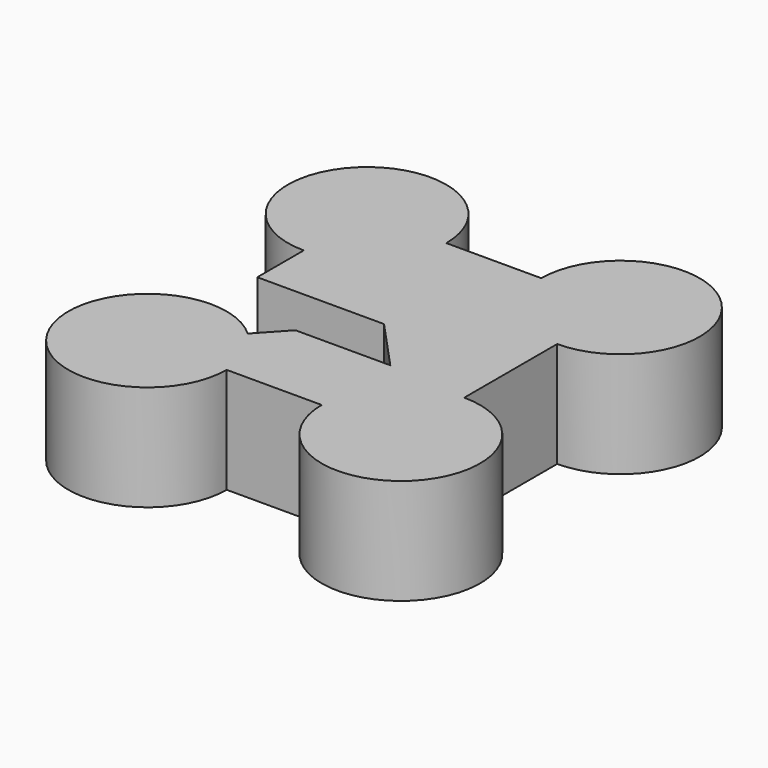
from build123d import *

# Parameters (mm, degrees)
F1_DEPTH = 25.4


with BuildPart() as f1:
    # F0 (on Top) → F1 (new body)
    with BuildSketch(Plane.XY):
        with BuildLine():
            Line((-30.48, 13.97), (-30.48, 0))
            Line((-30.48, 0), (-11.4207109466, 0))
            Line((-11.4207109466, 0), (-11.4207109466, 12.3724368588))
            Line((-11.4207109466, 12.3724368588), (-17.5587640429, 19.0219943798))
            ThreePointArc((-17.5587640429, 19.0219943798), (-23.5431241565, 15.277896023), (-30.48, 13.97))
        make_face()
        Polygon((-11.4207109466, 12.3724368588), (-11.4207109466, 0), (0, 0), align=None)
        with BuildLine():
            ThreePointArc((-17.5587640429, -19.0219943798), (-23.5431241565, -15.277896023), (-30.48, -13.97))
            Line((-30.48, -13.97), (-30.48, -33.02))
            Line((-30.48, -33.02), (-17.5587640429, -19.0219943798))
        make_face()
        with BuildLine():
            Line((-30.48, -33.02), (-30.48, -13.97))
            ThreePointArc((-30.48, -13.97), (-43.9503841816, -46.4903841816), (-11.43, -33.02))
            Line((-11.43, -33.02), (-30.48, -33.02))
        make_face()
        with BuildLine():
            ThreePointArc((-49.53, 33.02), (-43.9503841816, 19.5496158184), (-30.48, 13.97))
            Line((-30.48, 13.97), (-30.48, 33.02))
            Line((-30.48, 33.02), (-49.53, 33.02))
        make_face()
        with BuildLine():
            Line((-30.48, 33.02), (-30.48, 13.97))
            ThreePointArc((-30.48, 13.97), (-23.5431241565, 15.277896023), (-17.5587640429, 19.0219943798))
            Line((-17.5587640429, 19.0219943798), (-30.48, 33.02))
        make_face()
        Polygon((11.4207109466, 12.3724368588), (0, 0), (11.4207109466, 0), align=None)
        Polygon((-11.4207109466, 12.3724368588), (0, 0), (11.4207109466, 12.3724368588), align=None)
        Polygon((11.4207109466, 0), (0, 0), (11.4207109466, -12.3724368588), align=None)
        with BuildLine():
            Line((-17.5587640429, 19.0219943798), (-11.4207109466, 12.3724368588))
            Line((-11.4207109466, 12.3724368588), (11.4207109466, 12.3724368588))
            Line((11.4207109466, 12.3724368588), (17.5587640429, 19.0219943798))
            ThreePointArc((17.5587640429, 19.0219943798), (13.0293260161, 25.3795499145), (11.43, 33.02))
            Line((11.43, 33.02), (-11.43, 33.02))
            ThreePointArc((-11.43, 33.02), (-13.0293260161, 25.3795499145), (-17.5587640429, 19.0219943798))
        make_face()
        with BuildLine():
            Line((11.4207109466, -12.3724368588), (-11.4207109466, -12.3724368588))
            Line((-11.4207109466, -12.3724368588), (-17.5587640429, -19.0219943798))
            ThreePointArc((-17.5587640429, -19.0219943798), (-13.0293260161, -25.3795499145), (-11.43, -33.02))
            Line((-11.43, -33.02), (11.43, -33.02))
            ThreePointArc((11.43, -33.02), (13.0293260161, -25.3795499145), (17.5587640429, -19.0219943798))
            Line((17.5587640429, -19.0219943798), (11.4207109466, -12.3724368588))
        make_face()
        with BuildLine():
            Line((-17.5587640429, -19.0219943798), (-30.48, -33.02))
            Line((-30.48, -33.02), (-11.43, -33.02))
            ThreePointArc((-11.43, -33.02), (-13.0293260161, -25.3795499145), (-17.5587640429, -19.0219943798))
        make_face()
        with BuildLine():
            Line((-49.53, 33.02), (-30.48, 33.02))
            Line((-30.48, 33.02), (-11.43, 33.02))
            ThreePointArc((-11.43, 33.02), (-30.48, 52.07), (-49.53, 33.02))
        make_face()
        with BuildLine():
            Line((-11.43, 33.02), (-30.48, 33.02))
            Line((-30.48, 33.02), (-17.5587640429, 19.0219943798))
            ThreePointArc((-17.5587640429, 19.0219943798), (-13.0293260161, 25.3795499145), (-11.43, 33.02))
        make_face()
        with BuildLine():
            Line((11.4207109466, 12.3724368588), (11.4207109466, 0))
            Line((11.4207109466, 0), (30.48, 0))
            Line((30.48, 0), (30.48, 13.97))
            ThreePointArc((30.48, 13.97), (23.5431241565, 15.277896023), (17.5587640429, 19.0219943798))
            Line((17.5587640429, 19.0219943798), (11.4207109466, 12.3724368588))
        make_face()
        with BuildLine():
            Line((30.48, 0), (11.4207109466, 0))
            Line((11.4207109466, 0), (11.4207109466, -12.3724368588))
            Line((11.4207109466, -12.3724368588), (17.5587640429, -19.0219943798))
            ThreePointArc((17.5587640429, -19.0219943798), (23.5431241565, -15.277896023), (30.48, -13.97))
            Line((30.48, -13.97), (30.48, 0))
        make_face()
        with BuildLine():
            ThreePointArc((17.5587640429, -19.0219943798), (13.0293260161, -25.3795499145), (11.43, -33.02))
            Line((11.43, -33.02), (30.48, -33.02))
            Line((30.48, -33.02), (17.5587640429, -19.0219943798))
        make_face()
        with BuildLine():
            Line((30.48, -33.02), (11.43, -33.02))
            ThreePointArc((11.43, -33.02), (30.48, -52.07), (49.53, -33.02))
            ThreePointArc((49.53, -33.02), (43.9503841816, -19.5496158184), (30.48, -13.97))
            Line((30.48, -13.97), (30.48, -33.02))
        make_face()
        with BuildLine():
            ThreePointArc((11.43, 33.02), (13.0293260161, 25.3795499145), (17.5587640429, 19.0219943798))
            Line((17.5587640429, 19.0219943798), (30.48, 33.02))
            Line((30.48, 33.02), (11.43, 33.02))
        make_face()
        with BuildLine():
            Line((30.48, 33.02), (17.5587640429, 19.0219943798))
            ThreePointArc((17.5587640429, 19.0219943798), (23.5431241565, 15.277896023), (30.48, 13.97))
            Line((30.48, 13.97), (30.48, 33.02))
        make_face()
        with BuildLine():
            ThreePointArc((30.48, -13.97), (23.5431241565, -15.277896023), (17.5587640429, -19.0219943798))
            Line((17.5587640429, -19.0219943798), (30.48, -33.02))
            Line((30.48, -33.02), (30.48, -13.97))
        make_face()
        with BuildLine():
            ThreePointArc((49.53, 33.02), (30.48, 52.07), (11.43, 33.02))
            Line((11.43, 33.02), (30.48, 33.02))
            Line((30.48, 33.02), (49.53, 33.02))
        make_face()
        with BuildLine():
            Line((30.48, 33.02), (30.48, 13.97))
            ThreePointArc((30.48, 13.97), (43.9503841816, 19.5496158184), (49.53, 33.02))
            Line((49.53, 33.02), (30.48, 33.02))
        make_face()
    extrude(amount=F1_DEPTH)


solid = f1.part
